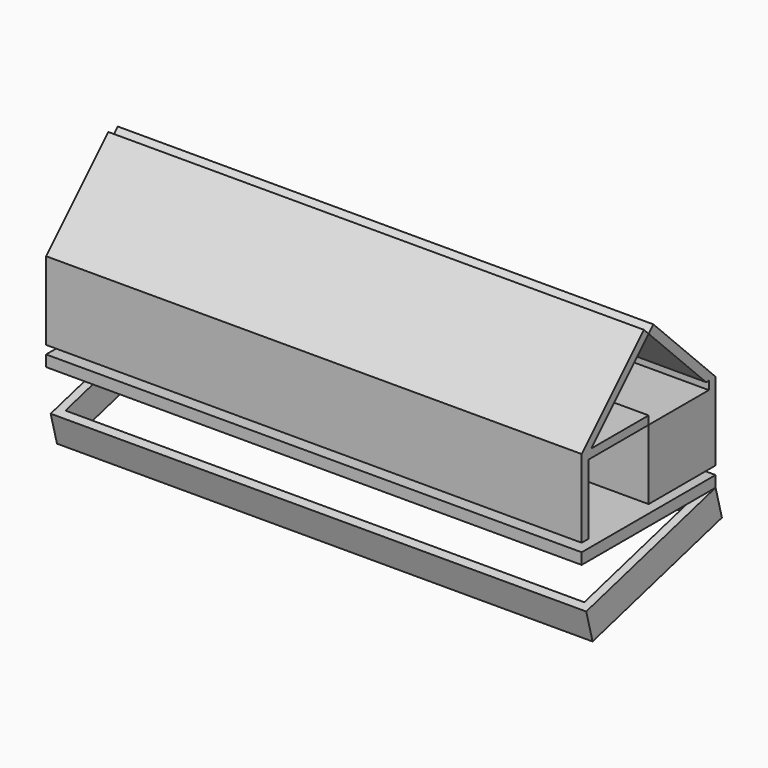
from build123d import *

# Parameters (mm, degrees)
F1_DEPTH = 2438.4
F2_W     = 2362.2
F2_H     = 685.8
F3_DEPTH = 203.2
F4_DEPTH = 2438.4
F0_W     = 342.9
F0_H     = 317.5
F0_W_2   = 38.1
F0_H_2   = 38.1


# Not quite as in the source:
# - a feature names something its author has since deleted; it is built from what else it names


with BuildPart() as f1:
    # F0 (on Right) → F1 (new body)
    with BuildSketch(Plane.YZ):
        Polygon((-914.8036036659, -223.8398379326), (-950.9606242668, -88.9), (-1686.996103899, -286.1201123681), (-1650.8390832982, -421.0599503007), align=None)
    extrude(amount=F1_DEPTH)

    # F2 (on face) → F3 (cut)
    with BuildSketch(Plane(origin=(0, -41.4772828265, 154.7953268685), x_dir=(1, 0, 0), z_dir=(0, -0.2588190451, 0.9659258263))):
        with Locations((1219.2, -1322.5664398729)):
            Rectangle(F2_W, F2_H)
    extrude(amount=-F3_DEPTH, mode=Mode.SUBTRACT)


with BuildPart() as f4:
    # F0 (on Right) → F4 (new body)
    with BuildSketch(Plane.YZ):
        Polygon((-950.9606242668, -88.9), (-950.9606242668, -38.1), (-1331.9606242668, -38.1), (-1712.9606242668, -38.1), (-1712.9606242668, -88.9), align=None)
    extrude(amount=F4_DEPTH)


with BuildPart() as f4b:
    # F0 (on Right) → F4, piece 2 (new body)
    with BuildSketch(Plane.YZ):
        with Locations((-1160.5106242668, 158.75)):
            Rectangle(F0_W, F0_H)
        with Locations((-970.0106242668, 158.75)):
            Rectangle(F0_W_2, F0_H)
        with Locations((-970.0106242668, 336.55)):
            Rectangle(F0_W_2, F0_H_2)
        Polygon((-989.0606242668, 355.6), (-950.9606242668, 355.6), (-1305.0198559036, 709.6592316368), (-1331.9606242668, 682.7184632736), (-1004.8421609932, 355.6), align=None)
    extrude(amount=F4_DEPTH)


with BuildPart() as f4c:
    # F0 (on Right) → F4, piece 3 (new body)
    with BuildSketch(Plane.YZ):
        with Locations((-1693.9106242668, 158.75)):
            Rectangle(F0_W_2, F0_H)
        with Locations((-1693.9106242668, 336.55)):
            Rectangle(F0_W_2, F0_H_2)
        Polygon((-1331.9606242668, 317.5), (-1331.9606242668, 355.6), (-1659.0790875403, 355.6), (-1674.8606242668, 355.6), (-1674.8606242668, 317.5), align=None)
        Polygon((-1659.0790875403, 355.6), (-1331.9606242668, 682.7184632736), (-1358.90139263, 709.6592316368), (-1712.9606242668, 355.6), (-1674.8606242668, 355.6), align=None)
    extrude(amount=F4_DEPTH)


solid = Compound([f1.part, f4.part, f4b.part, f4c.part])
